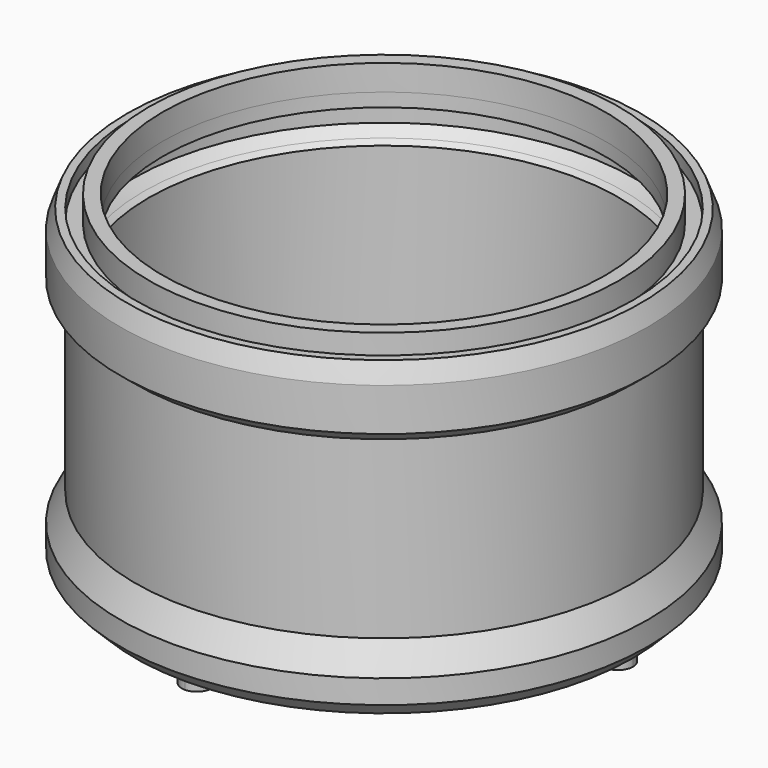
from build123d import *

# Parameters (mm, degrees)
F2_T            = 4.5
F4_DEPTH        = 2.5
F4_COPIES_COUNT = 4
F5_S5_R         = 5
F5_T6_DEPTH     = 125
F5_S7_R         = 5
F5_T8_DEPTH     = 125
F5_S9_R         = 5
F5_T10_DEPTH    = 125
F5_S11_R        = 5
F5_T12_DEPTH    = 125


# Not quite as in the source:
# - a fillet or chamfer that OpenCascade refuses, or shapes differently, is made with other operations: its cross-section is extruded or revolved along the edge and cut away or added
# - a pattern or mirror of a feature is missing from the dataset's text; its kind, count and spacing are read off the source's solid
# - a shell that OpenCascade refuses in one call is made with other operations: the cavity is built on its own and cut out


with BuildPart() as f1:
    # F0 (on Front) → F1 (revolve)
    with BuildSketch(Plane.XZ):
        Polygon((9.3241020494, -43.0905388618), (9.3241020494, 56.9094611382), (-63.8827484445, 56.9094611382), (-63.8827484445, 65.4041709328), (-68.4650088725, 65.4041709328), (-68.4650088725, 56.9094611382), (-73.0472693004, 56.9094611382), (-73.0472693004, 61.1568160355), (-75.6501782344, 61.1568160355), (-78.0099242383, 55.0157746972), (-78.0099242383, 40.8573164567), (-73.0472693004, 36.7660618934), (-73.0472693004, -21.2237248131), (-78.0099242383, -30.2868788943), (-78.0099242383, -43.0905388618), align=None)
    revolve(axis=Axis((9.3241020494, 0, 6.9094611382), (0, 0, 1)))

    # F2: shell of thickness 4.5, made by hand


with BuildPart() as f2_core1:
    # F2_t2: copy of F1
    add(f1.part)

    # the walls: a layer under each face that stays
    f2_faces = [f2_core1.faces().sort_by_distance(p)[0] for p in [
        (82.5309525433, 0, 61.1568160355),
        (-42.5353052318, 51.8594072813, 65.4041709328),
        (87.1132129713, 0, 61.1568160355),
        (-67.5558445438, 21.9656990266, 56.9094611382),
        (91.6954733993, 0, 59.0331385869),
        (-69.9852262155, 22.6598080757, 61.1568160355),
        (95.4782553352, 0, 58.0862953663),
        (96.6581283371, 0, 47.936545577),
        (94.1768008682, 0, 38.8116891751),
        (91.6954733993, 0, 7.7711685402),
        (94.1768008682, 0, -25.7553018537),
        (96.6581283371, 0, -36.688708878),
        (9.3241020494, 0, -43.0905388618),
    ]]
    thicken(f2_faces, amount=-F2_T, mode=Mode.SUBTRACT)

    # F2_s3 → F2_t4 (revolve, cut)
    with BuildSketch(Plane.XZ):
        Polygon((-68.5100088725, 56.9544611382), (-63.9650088725, 56.9094611382), (-63.9650088725, 52.4094611382), (-68.4650088725, 52.4094611382), align=None)
    revolve(axis=Axis((9.3241020494, 0, 56.9094611382), (0, 0, 1)), mode=Mode.SUBTRACT)

    # F2_s5 → F2_t6 (revolve, cut)
    with BuildSketch(Plane.XZ):
        Polygon((-73.0022693004, 56.9544611382), (-73.0472693004, 52.4094611382), (-77.5472693004, 52.4094611382), (-77.5472693004, 56.9094611382), align=None)
    revolve(axis=Axis((9.3241020494, 0, 56.9094611382), (0, 0, 1)), mode=Mode.SUBTRACT)

    # F2_s7 → F2_t8 (revolve, cut)
    with BuildSketch(Plane.XZ):
        Polygon((-73.1208943097, 36.731340015), (-70.1847683719, 40.2382497389), (-68.5472693004, 38.8882817011), (-68.5472693004, 36.7660618934), align=None)
    revolve(axis=Axis((9.3241020494, 0, 36.7660618934), (0, 0, 1)), mode=Mode.SUBTRACT)

    # F2_s9 → F2_t10 (revolve, cut)
    with BuildSketch(Plane.XZ):
        Polygon((-73.1317395514, -21.2021123331), (-68.5472693004, -21.2237248131), (-68.5472693004, -22.375090633), (-69.1002442047, -23.3849728075), align=None)
    revolve(axis=Axis((9.3241020494, 0, -21.2237248131), (0, 0, 1)), mode=Mode.SUBTRACT)


with BuildPart() as f1_1:
    add(f1.part)

    # what is left inside the walls is the cavity
    f2_cavity = [f2_core1.part.solids().sort_by_distance(p)[0] for p in [
        (87.150473, 0, 18.467158),
    ]]
    add(f2_cavity, mode=Mode.SUBTRACT)

    # F3 (on face) → F4 (join)
    with BuildSketch(Plane(origin=(0, 0, -43.0905388618), x_dir=(1, 0, 0), z_dir=(0, 0, -1))):
        with BuildLine():
            ThreePointArc((9.3241020494, 77.3856560126), (11.8241020494, 77.3452633101), (14.3214922181, 77.2241273697))
            ThreePointArc((14.3214922181, 77.2241273697), (14.323449549, 77.30488115), (14.3241020494, 77.3856560126))
            ThreePointArc((14.3241020494, 77.3856560126), (12.8596359554, 80.9211899185), (9.3241020494, 82.3856560126))
            Line((9.3241020494, 82.3856560126), (9.3241020494, 77.3856560126))
        make_face()
        with BuildLine():
            Line((9.3241020494, 77.3856560126), (9.3241020494, 72.3856560126))
            ThreePointArc((9.3241020494, 72.3856560126), (12.8020581148, 73.7934670411), (14.3214922181, 77.2241273697))
            ThreePointArc((14.3214922181, 77.2241273697), (11.8241020494, 77.3452633101), (9.3241020494, 77.3856560126))
        make_face()
        with BuildLine():
            ThreePointArc((4.3267118808, 77.2241273697), (5.8461459841, 73.7934670411), (9.3241020494, 72.3856560126))
            Line((9.3241020494, 72.3856560126), (9.3241020494, 77.3856560126))
            ThreePointArc((9.3241020494, 77.3856560126), (6.8241020494, 77.3452633101), (4.3267118808, 77.2241273697))
        make_face()
        with BuildLine():
            ThreePointArc((9.3241020494, 82.3856560126), (5.7319130779, 80.863612078), (4.3267118808, 77.2241273697))
            ThreePointArc((4.3267118808, 77.2241273697), (6.8241020494, 77.3452633101), (9.3241020494, 77.3856560126))
            Line((9.3241020494, 77.3856560126), (9.3241020494, 82.3856560126))
        make_face()
    f4 = extrude(amount=F4_DEPTH)

    # F4_copies: F4 ×4 about axis
    f4_copies_axis = Axis((9.324102, 0, 0), (0, 0, 1))
    for i in range(1, F4_COPIES_COUNT):
        add(f4.rotate(f4_copies_axis, i * 360 / F4_COPIES_COUNT))

    # F5: chamfer of 5 on 1 edges, made by hand


with BuildPart() as f5_tool2:
    # F5_s3 → F5_t4 (revolve)
    with BuildSketch(Plane.XZ):
        Polygon((-78.0099242383, -38.0905388618), (-73.0099242383, -43.0905388618), (-78.0099242383, -43.0905388618), align=None)
    revolve(axis=Axis((9.3241020494, 0, -43.0905388618), (0, 0, 1)))

    # F5_s5 → F5_t6 (cut, symmetric)
    with BuildSketch(Plane.XY.offset(-40.6)):
        with Locations((86.7097580126, 4.94e-08)):
            Circle(F5_S5_R)
    extrude(amount=F5_T6_DEPTH, both=True, mode=Mode.SUBTRACT)

    # F5_s7 → F5_t8 (cut, symmetric)
    with BuildSketch(Plane.XY.offset(-40.6)):
        with Locations((9.3241019506, 77.3856560126)):
            Circle(F5_S7_R)
    extrude(amount=F5_T8_DEPTH, both=True, mode=Mode.SUBTRACT)

    # F5_s9 → F5_t10 (cut, symmetric)
    with BuildSketch(Plane.XY.offset(-40.6)):
        with Locations((9.3241020494, -77.3856560126)):
            Circle(F5_S9_R)
    extrude(amount=F5_T10_DEPTH, both=True, mode=Mode.SUBTRACT)

    # F5_s11 → F5_t12 (cut, symmetric)
    with BuildSketch(Plane.XY.offset(-40.6)):
        with Locations((-68.0615540126, -4.94e-08)):
            Circle(F5_S11_R)
    extrude(amount=F5_T12_DEPTH, both=True, mode=Mode.SUBTRACT)


with BuildPart() as f1_2:
    add(f1_1.part)

    # F5_t1: cut F5_tool2
    add(f5_tool2.part, mode=Mode.SUBTRACT)


solid = f1_2.part
